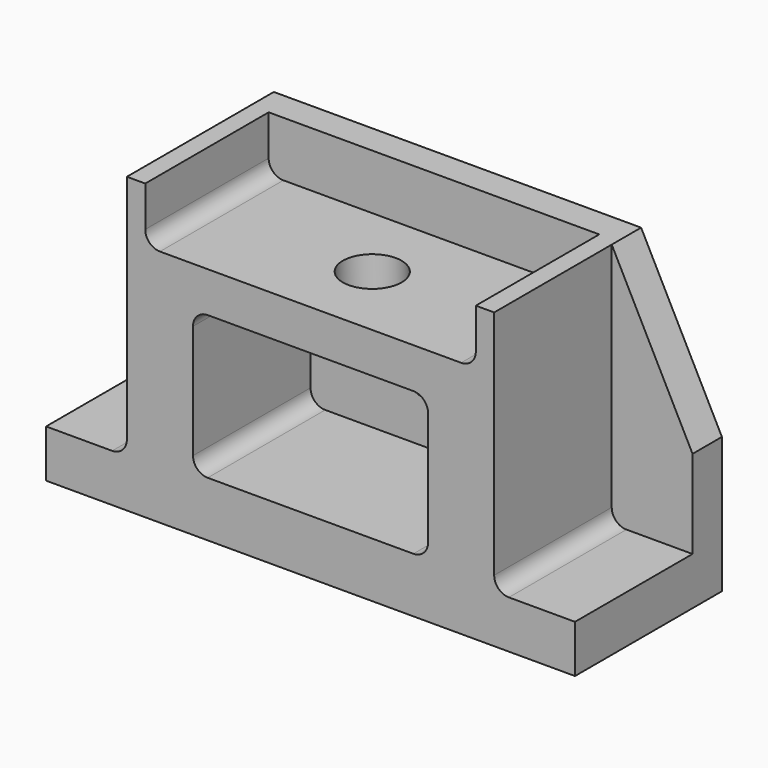
from build123d import *

# Parameters (mm, degrees)
F0_W      = 1440
F0_H      = 800
F1_DEPTH  = 500
F3_DEPTH  = 400
F5_DEPTH  = 400
F7_DEPTH  = 100.001
F9_DEPTH  = 100.001
F10_W     = 900
F10_H     = 420
F11_DEPTH = 150
F12_R     = 40
F13_R     = 80
F14_DEPTH = 150
F15_R     = 80
F16_DEPTH = 500.001


with BuildPart() as f1:
    # F0 (on Front) → F1 (new body)
    with BuildSketch(Plane.XZ):
        Rectangle(F0_W, F0_H)
    extrude(amount=F1_DEPTH)

    # F2 (on face) → F3 (cut)
    with BuildSketch(Plane.XZ.offset(500)):
        with BuildLine():
            Line((280, 140), (-280, 140))
            ThreePointArc((-280, 140), (-308.2842712475, 128.2842712475), (-320, 100))
            Line((-320, 100), (-320, -210))
            ThreePointArc((-320, -210), (-308.2842712475, -238.2842712475), (-280, -250))
            Line((-280, -250), (280, -250))
            ThreePointArc((280, -250), (308.2842712475, -238.2842712475), (320, -210))
            Line((320, -210), (320, 100))
            ThreePointArc((320, 100), (308.2842712475, 128.2842712475), (280, 140))
        make_face()
    extrude(amount=-F3_DEPTH, mode=Mode.SUBTRACT)

    # F4 (on face) → F5 (cut)
    with BuildSketch(Plane.XZ.offset(500)):
        with BuildLine():
            Line((-720, 400), (-720, -270))
            Line((-720, -270), (-540, -270))
            ThreePointArc((-540, -270), (-511.7157287525, -258.2842712475), (-500, -230))
            Line((-500, -230), (-500, 400))
            Line((-500, 400), (-720, 400))
        make_face()
        with BuildLine():
            Line((720, 400), (500, 400))
            Line((500, 400), (500, -230))
            ThreePointArc((500, -230), (511.7157287525, -258.2842712475), (540, -270))
            Line((540, -270), (720, -270))
            Line((720, -270), (720, 400))
        make_face()
    extrude(amount=-F5_DEPTH, mode=Mode.SUBTRACT)

    # F6 (on face) → F7 (cut, through all)
    with BuildSketch(Plane.XZ.offset(100)):
        Polygon((500, 400), (720, -30), (720, 400), align=None)
    extrude(amount=-F7_DEPTH, mode=Mode.SUBTRACT)

    # F8 (on face) → F9 (cut, through all)
    with BuildSketch(Plane.XZ.offset(100)):
        Polygon((-720, 400), (-720, -30), (-500, 400), align=None)
    extrude(amount=-F9_DEPTH, mode=Mode.SUBTRACT)

    # F10 (on face) → F11 (cut)
    with BuildSketch(Plane.XY.offset(400)):
        with Locations((0, -290)):
            Rectangle(F10_W, F10_H)
    extrude(amount=-F11_DEPTH, mode=Mode.SUBTRACT)

    # F12
    f12_edges = [f1.edges().sort_by_distance(p)[0] for p in [
        (-450, -290, 250),
        (450, -290, 250),
    ]]
    fillet(f12_edges, radius=F12_R)

    # F13 (on face) → F14 (cut)
    with BuildSketch(Plane.XY.offset(250)):
        with Locations((0, -290)):
            Circle(F13_R)
    extrude(amount=-F14_DEPTH, mode=Mode.SUBTRACT)

    # F15 (on face) → F16 (cut, through all)
    with BuildSketch(Plane(origin=(0, 0, 0), x_dir=(-1, 0, 0), z_dir=(0, 1, 0))):
        with Locations((0, -55)):
            Circle(F15_R)
    extrude(amount=-F16_DEPTH, mode=Mode.SUBTRACT)


solid = f1.part
